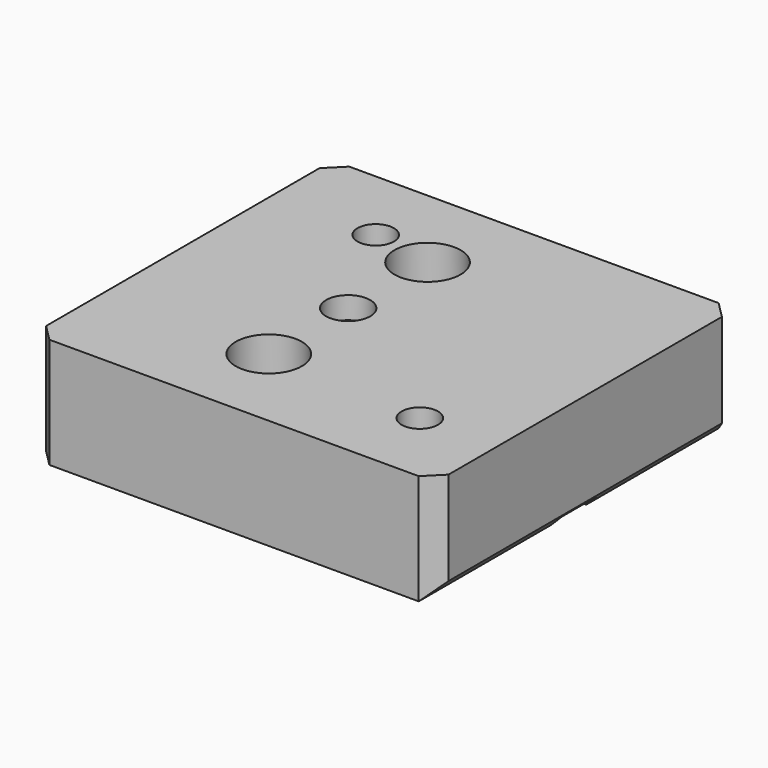
from build123d import *

# Parameters (mm, degrees)
F0_W        = 30
F0_H        = 30
F0_R        = 3
F0_R_2      = 1.65
F0_R_3      = 2
F0_R_4      = 1.5
F1_DEPTH    = 10
F2_DEPTH    = 12
F3_DEPTH    = 4
F4_R        = 2
F5_DEPTH    = 8
F6_DEPTH    = 1
F7_DEPTH    = 4.5
F8_DEPTH    = 2
F9_DEPTH    = 2
F10_DEPTH   = 2
F11_C1_SIZE = 1.5
F11_C2_SIZE = 1.5
F11_C3_SIZE = 1.5
F11_C4_SIZE = 1.5
F11_C5_SIZE = 1.5
F12_R       = 1.65
F13_DEPTH   = 8


# Not quite as in the source:
# - a feature names something its author has since deleted; it is built from what else it names


with BuildPart() as f1:
    # F0 (on Top) → F1 (new body)
    with BuildSketch(Plane.XY):
        with Locations((15, -15)):
            Rectangle(F0_W, F0_H)
        with Locations((15, -24)):
            Circle(F0_R, mode=Mode.SUBTRACT)
        with Locations((6, -15)):
            Circle(F0_R, mode=Mode.SUBTRACT)
        with Locations((9.5, -5)):
            Circle(F0_R_2, mode=Mode.SUBTRACT)
        with Locations((15, -15)):
            Circle(F0_R_3, mode=Mode.SUBTRACT)
        with Locations((24, -15)):
            Circle(F0_R, mode=Mode.SUBTRACT)
        with Locations((15, -6)):
            Circle(F0_R, mode=Mode.SUBTRACT)
        with Locations((15, -6)):
            Circle(F0_R)
        with Locations((15, -6)):
            Circle(F0_R_4, mode=Mode.SUBTRACT)
        with Locations((15, -24)):
            Circle(F0_R)
        with Locations((15, -24)):
            Circle(F0_R_4, mode=Mode.SUBTRACT)
        with Locations((24, -15)):
            Circle(F0_R)
        with Locations((24, -15)):
            Circle(F0_R_4, mode=Mode.SUBTRACT)
        with Locations((6, -15)):
            Circle(F0_R)
        with Locations((6, -15)):
            Circle(F0_R_4, mode=Mode.SUBTRACT)
        with Locations((15, -15)):
            Circle(F0_R_3)
        with Locations((9.5, -5)):
            Circle(F0_R_2)
        with Locations((6, -15)):
            Circle(F0_R_4)
        with Locations((24, -15)):
            Circle(F0_R_4)
    extrude(amount=-F1_DEPTH)

    # F0 (on Top) → F2 (cut)
    with BuildSketch(Plane.XY):
        with Locations((15, -15)):
            Circle(F0_R_3)
    extrude(amount=-F2_DEPTH, mode=Mode.SUBTRACT)

    # F0 (on Top) → F3 (cut)
    with BuildSketch(Plane.XY):
        with Locations((15, -24)):
            Circle(F0_R)
        with Locations((15, -24)):
            Circle(F0_R_4, mode=Mode.SUBTRACT)
        with Locations((15, -6)):
            Circle(F0_R)
        with Locations((15, -6)):
            Circle(F0_R_4, mode=Mode.SUBTRACT)
    extrude(amount=-F3_DEPTH, mode=Mode.SUBTRACT)

    # F4 (on face) → F5 (cut)
    with BuildSketch(Plane(origin=(0, 0, -10), x_dir=(1, 0, 0), z_dir=(0, 0, -1))):
        with BuildLine():
            ThreePointArc((19.6, 13.0404082058), (18, 15), (19.6, 16.9595917942))
            ThreePointArc((19.6, 16.9595917942), (10, 15), (19.6, 13.0404082058))
        make_face()
        with Locations((15, 15)):
            Circle(F4_R, mode=Mode.SUBTRACT)
        with BuildLine():
            ThreePointArc((19.6, 13.0404082058), (19.8989794856, 14), (20, 15))
            ThreePointArc((20, 15), (19.8989794856, 16), (19.6, 16.9595917942))
            ThreePointArc((19.6, 16.9595917942), (18, 15), (19.6, 13.0404082058))
        make_face()
    extrude(amount=-F5_DEPTH, mode=Mode.SUBTRACT)

    # F4 (on face) → F6 (cut)
    with BuildSketch(Plane(origin=(0, 0, -10), x_dir=(1, 0, 0), z_dir=(0, 0, -1))):
        with BuildLine():
            ThreePointArc((19.6, 16.9595917942), (19.8989794856, 16), (20, 15))
            ThreePointArc((20, 15), (19.8989794856, 14), (19.6, 13.0404082058))
            ThreePointArc((19.6, 13.0404082058), (19.798982076, 13.010127694), (20, 13))
            Line((20, 13), (30, 13))
            Line((30, 13), (30, 17))
            Line((30, 17), (20, 17))
            ThreePointArc((20, 17), (19.798982076, 16.989872306), (19.6, 16.9595917942))
        make_face()
    extrude(amount=-F6_DEPTH, mode=Mode.SUBTRACT)

    # F7 (add): a face of the model
    f7_faces = [f1.faces().sort_by_distance(p)[0] for p in [
        (30, -15, -4.9391891892),
    ]]
    extrude(f7_faces, amount=F7_DEPTH)

    # F8 (add): a face of the model
    f8_faces = [f1.faces().sort_by_distance(p)[0] for p in [
        (17.25, 0, -5),
    ]]
    extrude(f8_faces, amount=F8_DEPTH)

    # F9 (add): a face of the model
    f9_faces = [f1.faces().sort_by_distance(p)[0] for p in [
        (17.25, -30, -5),
    ]]
    extrude(f9_faces, amount=F9_DEPTH)

    # F10 (add): a face of the model
    f10_faces = [f1.faces().sort_by_distance(p)[0] for p in [
        (34.5, -15, -4.9464285714),
    ]]
    extrude(f10_faces, amount=F10_DEPTH)

    # F11: chamfer of 1.5 on 6 edges, made by hand

    # F11_c1
    f11_c1_edges = [f1.edges().sort_by_distance(p)[0] for p in [
        (36.5, -5.5, -10),
    ]]
    chamfer(f11_c1_edges, length=F11_C1_SIZE)

    # F11_c2
    f11_c2_edges = [f1.edges().sort_by_distance(p)[0] for p in [
        (0, -32, -5),
    ]]
    chamfer(f11_c2_edges, length=F11_C2_SIZE)

    # F11_c3
    f11_c3_edges = [f1.edges().sort_by_distance(p)[0] for p in [
        (36.5, -32, -4.25),
    ]]
    chamfer(f11_c3_edges, length=F11_C3_SIZE)

    # F11_c4
    f11_c4_edges = [f1.edges().sort_by_distance(p)[0] for p in [
        (0, 2, -5),
    ]]
    chamfer(f11_c4_edges, length=F11_C4_SIZE)

    # F11_c5
    f11_c5_edges = [f1.edges().sort_by_distance(p)[0] for p in [
        (36.5, 2, -4.25),
    ]]
    chamfer(f11_c5_edges, length=F11_C5_SIZE)

    # F0 (on Top) + F12 (on face) → F13 (cut)
    with BuildSketch(Plane.XY):
        with Locations((9.5, -5)):
            Circle(F0_R_2)
    with BuildSketch(Plane.XY):
        with Locations((29.5, -25)):
            Circle(F12_R)
    extrude(amount=-F13_DEPTH, mode=Mode.SUBTRACT)


solid = f1.part
